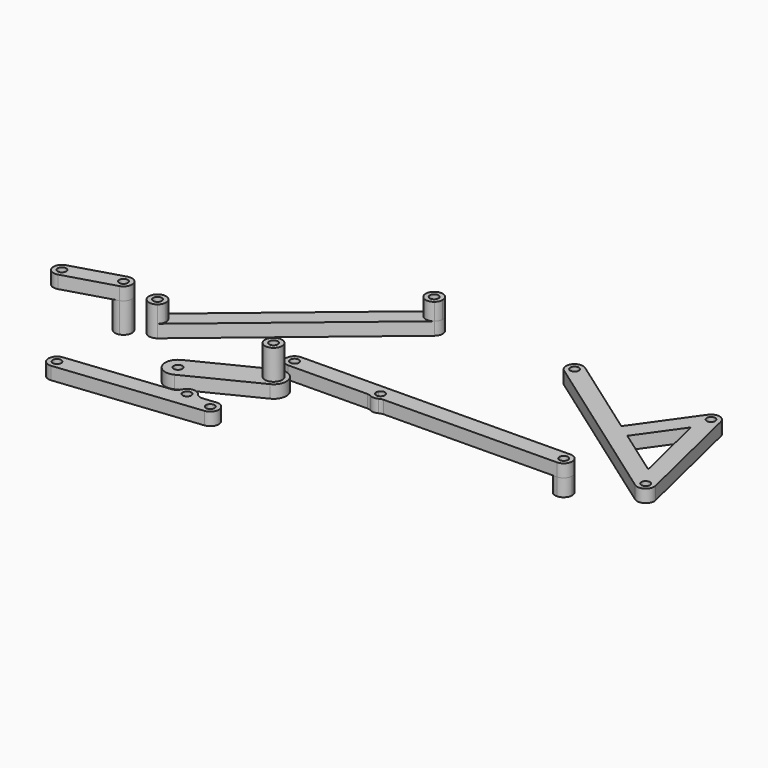
from build123d import *
from build123d import SkipClean  # not in build123d's __all__

# Parameters (mm, degrees)
F1_DEPTH  = 7.5
F2_R      = 5
F4_DEPTH  = 7.5
F5_R      = 5
F7_DEPTH  = 7.5
F8_R      = 2.5
F9_DEPTH  = 7.5
F11_DEPTH = 7.5
F12_R     = 2.5
F13_DEPTH = 10
F14_R     = 2.5
F15_DEPTH = 10
F16_R     = 2.5
F17_DEPTH = 17.5
F18_R     = 2.5
F19_DEPTH = 10
F20_R     = 5
F20_R_2   = 2.5
F21_DEPTH = 17.5


with BuildPart() as f1:
    # F0 (on Top) → F1 (new body)
    with BuildSketch(Plane.XY):
        with BuildLine():
            ThreePointArc((-1.6252031285, -41.1984268842), (-3.9906722267, -43.6948045472), (-6.6107242777, -41.4670988347))
            Line((-6.6107242777, -41.4670988347), (-14.4692804683, -42.316568018))
            ThreePointArc((-14.4692804683, -42.316568018), (-15.5453055293, -45.9890101187), (-18.9029788583, -47.8249542167))
            Line((-18.9029788583, -47.8249542167), (-3.5878592274, -46.1694691825))
            ThreePointArc((-3.5878592274, -46.1694691825), (0.8458391698, -40.661082983), (-4.6625470297, -36.2273845858))
            Line((-4.6625470297, -36.2273845858), (-15.3535819474, -37.3830300351))
            Line((-15.3535819474, -37.3830300351), (-15.0474170603, -39.0658729224))
            Line((-15.0474170603, -39.0658729224), (-6.5788708842, -40.7193501214))
            ThreePointArc((-6.5788708842, -40.7193501214), (-3.8845471388, -38.7100369038), (-1.6252031285, -41.1984268842))
        make_face()
        with BuildLine():
            ThreePointArc((-18.9029788583, -47.8249542167), (-15.5453055293, -45.9890101187), (-14.4692804683, -42.316568018))
            Line((-14.4692804683, -42.316568018), (-19.4403227667, -42.8539119191))
            Line((-19.4403227667, -42.8539119191), (-24.4243816475, -43.3926628454))
            Line((-24.4243816475, -43.3926628454), (-24.3595727591, -43.7488865063))
            ThreePointArc((-24.3595727591, -43.7488865063), (-22.432622422, -46.8596756132), (-18.9029788583, -47.8249542167))
        make_face()
        with BuildLine():
            Line((-17.8630008002, -38.516132339), (-15.0474170603, -39.0658729224))
            Line((-15.0474170603, -39.0658729224), (-15.3535819474, -37.3830300351))
            Line((-15.3535819474, -37.3830300351), (-15.3974185634, -37.1420809891))
            ThreePointArc((-15.3974185634, -37.1420809891), (-20.9754157833, -33.0806403303), (-25.2989118261, -38.4580686356))
            Line((-25.2989118261, -38.4580686356), (-87.3721108551, -45.1678596456))
            ThreePointArc((-87.3721108551, -45.1678596456), (-91.8058092522, -50.6762458451), (-86.2974230527, -55.1099442423))
            Line((-86.2974230527, -55.1099442423), (-18.9029788583, -47.8249542167))
            ThreePointArc((-18.9029788583, -47.8249542167), (-22.432622422, -46.8596756132), (-24.3595727591, -43.7488865063))
            Line((-24.3595727591, -43.7488865063), (-24.4243816475, -43.3926628454))
            Line((-24.4243816475, -43.3926628454), (-84.3492458047, -49.8702299933))
            ThreePointArc((-84.3492458047, -49.8702299933), (-84.3383892909, -50.0043710421), (-84.3347669539, -50.1389019439))
            ThreePointArc((-84.3347669539, -50.1389019439), (-89.3246527435, -50.3635544639), (-84.3751419577, -49.6914146503))
            Line((-84.3751419577, -49.6914146503), (-25.2359185483, -38.9320301634))
            Line((-25.2359185483, -38.9320301634), (-22.7762935521, -38.4845428698))
            ThreePointArc((-22.7762935521, -38.4845428698), (-22.7985582034, -38.337428307), (-22.8120316405, -38.1892497802))
            ThreePointArc((-22.8120316405, -38.1892497802), (-20.5853405064, -35.5515344271), (-17.8464232598, -37.6524932574))
            ThreePointArc((-17.8464232598, -37.6524932574), (-17.8241183317, -37.8441997236), (-17.8166685559, -38.0370555762))
            ThreePointArc((-17.8166685559, -38.0370555762), (-17.8282785754, -38.2777115659), (-17.8630008002, -38.516132339))
        make_face()
        with BuildLine():
            Line((-84.3492458047, -49.8702299933), (-24.4243816475, -43.3926628454))
            Line((-24.4243816475, -43.3926628454), (-25.2359185483, -38.9320301634))
            Line((-25.2359185483, -38.9320301634), (-84.3751419577, -49.6914146503))
            ThreePointArc((-84.3751419577, -49.6914146503), (-84.3605779289, -49.7805882986), (-84.3492458047, -49.8702299933))
        make_face()
        with BuildLine():
            Line((-24.4243816475, -43.3926628454), (-19.4403227667, -42.8539119191))
            Line((-19.4403227667, -42.8539119191), (-19.8691812623, -40.4966805725))
            ThreePointArc((-19.8691812623, -40.4966805725), (-21.7394647701, -40.09269439), (-22.7762935521, -38.4845428698))
            Line((-22.7762935521, -38.4845428698), (-25.2359185483, -38.9320301634))
            Line((-25.2359185483, -38.9320301634), (-24.4243816475, -43.3926628454))
        make_face()
        with BuildLine():
            Line((-19.4403227667, -42.8539119191), (-14.4692804683, -42.316568018))
            ThreePointArc((-14.4692804683, -42.316568018), (-14.4919447166, -42.1372846285), (-14.5210727742, -41.958937332))
            Line((-14.5210727742, -41.958937332), (-15.0474170603, -39.0658729224))
            Line((-15.0474170603, -39.0658729224), (-17.8630008002, -38.516132339))
            ThreePointArc((-17.8630008002, -38.516132339), (-18.560303565, -39.8161514193), (-19.8691812623, -40.4966805725))
            Line((-19.8691812623, -40.4966805725), (-19.4403227667, -42.8539119191))
        make_face()
        with BuildLine():
            Line((-14.4692804683, -42.316568018), (-6.6107242777, -41.4670988347))
            ThreePointArc((-6.6107242777, -41.4670988347), (-6.6229378611, -41.0920257285), (-6.5788708842, -40.7193501214))
            Line((-6.5788708842, -40.7193501214), (-15.0474170603, -39.0658729224))
            Line((-15.0474170603, -39.0658729224), (-14.5210727742, -41.958937332))
            ThreePointArc((-14.5210727742, -41.958937332), (-14.4919447166, -42.1372846285), (-14.4692804683, -42.316568018))
        make_face()
    extrude(amount=F1_DEPTH)

    # F2
    f2_edges = [f1.edges().sort_by_distance(p)[0] for p in [
        (-15.353582, -37.38303, 3.75),
        (-25.298912, -38.458069, 3.75),
    ]]
    fillet(f2_edges, radius=F2_R)


with BuildPart() as f4:
    # F3 (on Top) → F4 (new body)
    with BuildSketch(Plane.XY):
        with BuildLine():
            ThreePointArc((0.3729692735, 18.0101927138), (-4.6268408802, 18.0424809595), (0.3730047678, 18.0687030944))
            Line((0.3730047678, 18.0687030944), (43.7480600824, 18.5500000326))
            ThreePointArc((43.7480600824, 18.5500000326), (45.173207574, 22.1015652772), (48.6922749028, 23.6051696781))
            Line((48.6922749028, 23.6051696781), (-2.1823187693, 23.0406565959))
            ThreePointArc((-2.1823187693, 23.0406565959), (-7.1265335562, 17.9854869508), (-2.0713639111, 13.0412721639))
            Line((-2.0713639111, 13.0412721639), (45.5774592227, 13.5699915515))
            ThreePointArc((45.5774592227, 13.5699915515), (44.2716236478, 15.240737181), (43.7756797378, 17.3024445185))
            Line((43.7756797378, 17.3024445185), (43.7717936651, 17.4759705915))
            Line((43.7717936651, 17.4759705915), (0.3729692735, 18.0101927138))
        make_face()
        with BuildLine():
            ThreePointArc((48.6922749028, 23.6051696781), (45.173207574, 22.1015652772), (43.7480600824, 18.5500000326))
            Line((43.7480600824, 18.5500000326), (46.5634398285, 18.5812399617))
            ThreePointArc((46.5634398285, 18.5812399617), (48.7466876828, 19.9142362969), (50.9589766417, 18.6300135804))
            Line((50.9589766417, 18.6300135804), (53.7477634707, 18.66095843))
            Line((53.7477634707, 18.66095843), (53.746498958, 18.7174231321))
            ThreePointArc((53.746498958, 18.7174231321), (52.2235967035, 22.1997097401), (48.6922749028, 23.6051696781))
        make_face()
        with BuildLine():
            Line((46.2746157836, 17.445161855), (43.7717936651, 17.4759705915))
            Line((43.7717936651, 17.4759705915), (43.7756797378, 17.3024445185))
            ThreePointArc((43.7756797378, 17.3024445185), (44.2716236478, 15.240737181), (45.5774592227, 13.5699915515))
            Line((45.5774592227, 13.5699915515), (52.0559121057, 13.6418775586))
            ThreePointArc((52.0559121057, 13.6418775586), (53.3474796541, 15.3927117005), (53.773173057, 17.5263358594))
            Line((53.773173057, 17.5263358594), (51.2737997272, 17.4703630242))
            ThreePointArc((51.2737997272, 17.4703630242), (51.2742697249, 17.4423783605), (51.2744263974, 17.4143901889))
            ThreePointArc((51.2744263974, 17.4143901889), (48.7590402729, 14.9144375359), (46.2746157836, 17.445161855))
        make_face()
        with BuildLine():
            Line((154.1643564376, 24.775505705), (48.6922749028, 23.6051696781))
            ThreePointArc((48.6922749028, 23.6051696781), (52.2235967035, 22.1997097401), (53.746498958, 18.7174231321))
            Line((53.746498958, 18.7174231321), (53.7477634707, 18.66095843))
            Line((53.7477634707, 18.66095843), (151.7199877587, 19.7480747745))
            ThreePointArc((151.7199877587, 19.7480747745), (154.205964296, 22.2757750157), (156.7198338667, 19.775813489))
            ThreePointArc((156.7198338667, 19.775813489), (154.2478220383, 17.2759701615), (151.7204605369, 19.7198406538))
            Line((151.7204605369, 19.7198406538), (53.773173057, 17.5263358594))
            ThreePointArc((53.773173057, 17.5263358594), (53.3474796541, 15.3927117005), (52.0559121057, 13.6418775586))
            Line((52.0559121057, 13.6418775586), (154.2753112958, 14.776121273))
            ThreePointArc((154.2753112958, 14.776121273), (159.2195260827, 19.8312909181), (154.1643564376, 24.775505705))
        make_face()
        with BuildLine():
            Line((52.0559121057, 13.6418775586), (45.5774592227, 13.5699915515))
            ThreePointArc((45.5774592227, 13.5699915515), (48.8299038265, 12.4146979729), (52.0559121057, 13.6418775586))
        make_face()
        with BuildLine():
            Line((151.7199877587, 19.7480747745), (53.7477634707, 18.66095843))
            Line((53.7477634707, 18.66095843), (53.773173057, 17.5263358594))
            Line((53.773173057, 17.5263358594), (151.7204605369, 19.7198406538))
            ThreePointArc((151.7204605369, 19.7198406538), (151.7201842836, 19.7339570466), (151.7199877587, 19.7480747745))
        make_face()
        with BuildLine():
            Line((46.5634398285, 18.5812399617), (43.7480600824, 18.5500000326))
            ThreePointArc((43.7480600824, 18.5500000326), (43.7484531322, 18.5217645769), (43.7490056388, 18.4935317913))
            Line((43.7490056388, 18.4935317913), (43.7717936651, 17.4759705915))
            Line((43.7717936651, 17.4759705915), (46.2746157836, 17.445161855))
            ThreePointArc((46.2746157836, 17.445161855), (46.3515002965, 18.0303683622), (46.5634398285, 18.5812399617))
        make_face()
        with BuildLine():
            Line((43.7480600824, 18.5500000326), (0.3730047678, 18.0687030944))
            ThreePointArc((0.3730047678, 18.0687030944), (0.3731201865, 18.0548339506), (0.3731586598, 18.0409643799))
            ThreePointArc((0.3731586598, 18.0409643799), (0.3731113128, 18.0255782555), (0.3729692735, 18.0101927138))
            Line((0.3729692735, 18.0101927138), (43.7717936651, 17.4759705915))
            Line((43.7717936651, 17.4759705915), (43.7490056388, 18.4935317913))
            ThreePointArc((43.7490056388, 18.4935317913), (43.7484531322, 18.5217645769), (43.7480600824, 18.5500000326))
        make_face()
        with BuildLine():
            Line((53.7477634707, 18.66095843), (50.9589766417, 18.6300135804))
            ThreePointArc((50.9589766417, 18.6300135804), (51.1870976069, 18.0693845666), (51.2737997272, 17.4703630242))
            Line((51.2737997272, 17.4703630242), (53.773173057, 17.5263358594))
            Line((53.773173057, 17.5263358594), (53.7477634707, 18.66095843))
        make_face()
    extrude(amount=F4_DEPTH)

    # F5
    f5_edges = [f4.edges().sort_by_distance(p)[0] for p in [
        (45.577459, 13.569992, 3.75),
        (52.055912, 13.641878, 3.75),
    ]]
    fillet(f5_edges, radius=F5_R)

    # F14 (on face) → F15 (join)
    with BuildSketch(Plane(origin=(0, 0, 0), x_dir=(1, 0, 0), z_dir=(0, 0, -1))):
        with BuildLine():
            ThreePointArc((154.2753112958, -14.776121273), (149.2201416507, -19.7203360599), (154.1643564376, -24.775505705))
            ThreePointArc((154.1643564376, -24.775505705), (157.7356988282, -23.3309075205), (159.2198338667, -19.775813489))
            ThreePointArc((159.2198338667, -19.775813489), (157.7749278982, -16.2599485275), (154.2753112958, -14.776121273))
        make_face()
        with Locations((154.2198338667, -19.775813489)):
            Circle(F14_R, mode=Mode.SUBTRACT)
    extrude(amount=F15_DEPTH)


with BuildPart() as f7:
    # F6 (on Top) → F7 (new body)
    with BuildSketch(Plane.XY):
        with BuildLine():
            ThreePointArc((23.0980938211, 88.9733356379), (23.7370777778, 96.0154730622), (16.6949403535, 96.6544570189))
            Line((16.6949403535, 96.6544570189), (-80.5939894362, 15.5522432611))
            ThreePointArc((-80.5939894362, 15.5522432611), (-81.2329733929, 8.5101058368), (-74.1908359686, 7.8711218801))
            Line((-74.1908359686, 7.8711218801), (23.0980938211, 88.9733356379))
        make_face()
        with BuildLine():
            ThreePointArc((-74.8924127024, 11.7116825706), (-79.743019099, 10.8604190577), (-75.4721323571, 13.3124709375))
            ThreePointArc((-75.4721323571, 13.3124709375), (-75.0418063058, 12.5629460835), (-74.8924127024, 11.7116825706))
        make_face(mode=Mode.SUBTRACT)
        with BuildLine():
            ThreePointArc((22.3965170873, 92.8138963284), (20.7477806002, 90.4632899318), (17.976236742, 91.2131079615))
            ThreePointArc((17.976236742, 91.2131079615), (19.0452535744, 95.164502725), (22.3965170873, 92.8138963284))
        make_face(mode=Mode.SUBTRACT)
    extrude(amount=F7_DEPTH)

    # F12 (on face) → F13 (join)
    with BuildSketch(Plane.XY.offset(7.5)):
        with BuildLine():
            ThreePointArc((24.8965170873, 92.8138963284), (22.016908128, 97.3420241794), (16.6949403535, 96.6544570189))
            ThreePointArc((16.6949403535, 96.6544570189), (16.0559563968, 89.6123195946), (23.0980938211, 88.9733356379))
            ThreePointArc((23.0980938211, 88.9733356379), (24.4246449382, 90.6935052877), (24.8965170873, 92.8138963284))
        make_face()
        with Locations((19.8965170873, 92.8138963284)):
            Circle(F12_R, mode=Mode.SUBTRACT)
    extrude(amount=F13_DEPTH)

    # F18 (on face) → F19 (join)
    with BuildSketch(Plane.XY.offset(7.5)):
        with BuildLine():
            ThreePointArc((-80.5939894362, 15.5522432611), (-81.2329733929, 8.5101058368), (-74.1908359686, 7.8711218801))
            ThreePointArc((-74.1908359686, 7.8711218801), (-72.8642848515, 9.5912915299), (-72.3924127024, 11.7116825706))
            ThreePointArc((-72.3924127024, 11.7116825706), (-75.2720216617, 16.2398104216), (-80.5939894362, 15.5522432611))
        make_face()
        with Locations((-77.3924127024, 11.7116825706)):
            Circle(F18_R, mode=Mode.SUBTRACT)
    extrude(amount=F19_DEPTH)


with BuildPart() as f7b:
    # F6 (on Top) → F7, piece 2 (new body)
    with BuildSketch(Plane.XY):
        with BuildLine():
            ThreePointArc((-143.2768418385, 27.0090536761), (-146.6393941629, 20.7886644707), (-140.4190049575, 17.4261121464))
            Line((-140.4190049575, 17.4261121464), (-111.2633845005, 26.1209379651))
            ThreePointArc((-111.2633845005, 26.1209379651), (-107.9008321762, 32.3413271705), (-114.1212213815, 35.7038794948))
            Line((-114.1212213815, 35.7038794948), (-143.2768418385, 27.0090536761))
        make_face()
        with BuildLine():
            ThreePointArc((-139.347923398, 22.2175829113), (-144.3217199192, 21.8565693769), (-139.4521880156, 22.9320421315))
            ThreePointArc((-139.4521880156, 22.9320421315), (-139.3741268769, 22.5785964456), (-139.347923398, 22.2175829113))
        make_face(mode=Mode.SUBTRACT)
        with BuildLine():
            ThreePointArc((-110.192302941, 30.9124087299), (-112.3312894067, 28.4386122088), (-115.0880383234, 30.1979495097))
            ThreePointArc((-115.0880383234, 30.1979495097), (-113.0533164754, 33.3862052511), (-110.192302941, 30.9124087299))
        make_face(mode=Mode.SUBTRACT)
    extrude(amount=F7_DEPTH)

    # F16 (on face) → F17 (join)
    with BuildSketch(Plane(origin=(0, 0, 0), x_dir=(1, 0, 0), z_dir=(0, 0, -1))):
        with BuildLine():
            ThreePointArc((-111.2633845005, -26.1209379651), (-117.4837737059, -29.4834902894), (-114.1212213815, -35.7038794948))
            ThreePointArc((-114.1212213815, -35.7038794948), (-109.7043765867, -34.9214355571), (-107.692302941, -30.9124087299))
            ThreePointArc((-107.692302941, -30.9124087299), (-108.6832761138, -27.9244823756), (-111.2633845005, -26.1209379651))
        make_face()
        with Locations((-112.692302941, -30.9124087299)):
            Circle(F16_R, mode=Mode.SUBTRACT)
    with SkipClean():  # cleaning this boolean's faces spoils the solid; the shape is the same uncleaned
        extrude(amount=F17_DEPTH)


with BuildPart() as f9:
    # F8 (on Top) → F9 (new body)
    with BuildSketch(Plane.XY):
        with BuildLine():
            ThreePointArc((102.7963197006, 96.9999852765), (98.0322393826, 93.5173869112), (99.9046646538, 87.9210509443))
            Line((99.9046646538, 87.9210509443), (196.2528462269, 19.6149425153))
            ThreePointArc((196.2528462269, 19.6149425153), (195.002467233, 20.8934023144), (194.2819356808, 22.5300884078))
            Line((194.2819356808, 22.5300884078), (191.1861989539, 35.4650492124))
            Line((191.1861989539, 35.4650492124), (162.9887393202, 55.4556572728))
            Line((162.9887393202, 55.4556572728), (154.8587189983, 61.2194406735))
            Line((154.8587189983, 61.2194406735), (105.6881911573, 96.078919611))
            ThreePointArc((105.6881911573, 96.078919611), (104.3138295391, 96.7641738006), (102.7963197006, 96.9999852765))
        make_face()
        with Locations((102.7964279056, 91.9999852777)):
            Circle(F8_R, mode=Mode.SUBTRACT)
        with BuildLine():
            ThreePointArc((194.2819356808, 22.5300884078), (195.002467233, 20.8934023144), (196.2528462269, 19.6149425153))
            ThreePointArc((196.2528462269, 19.6149425153), (201.9450840129, 19.551734603), (204.0072832766, 24.8576652895))
            ThreePointArc((204.0072832766, 24.8576652895), (203.2867517243, 26.4943513829), (202.0363727305, 27.772811182))
            Line((202.0363727305, 27.772811182), (191.1861989539, 35.4650492124))
            Line((191.1861989539, 35.4650492124), (194.2819356808, 22.5300884078))
        make_face()
        with Locations((199.1446094787, 23.6938768487)):
            Circle(F8_R, mode=Mode.SUBTRACT)
        with BuildLine():
            ThreePointArc((202.0363727305, 27.772811182), (203.2867517243, 26.4943513829), (204.0072832766, 24.8576652895))
            Line((204.0072832766, 24.8576652895), (187.6591016847, 93.165504998))
            ThreePointArc((187.6591016847, 93.165504998), (187.6552696367, 90.8220314934), (186.5840700208, 88.737705671))
            Line((186.5840700208, 88.737705671), (180.4927420797, 80.1456721912))
            Line((180.4927420797, 80.1456721912), (191.1861989539, 35.4650492124))
            Line((191.1861989539, 35.4650492124), (202.0363727305, 27.772811182))
        make_face()
        with BuildLine():
            Line((178.5286055467, 94.6066527316), (154.8587189983, 61.2194406735))
            Line((154.8587189983, 61.2194406735), (162.9887393202, 55.4556572728))
            Line((162.9887393202, 55.4556572728), (180.4927420797, 80.1456721912))
            Line((180.4927420797, 80.1456721912), (177.9337540889, 90.8379281163))
            ThreePointArc((177.9337540889, 90.8379281163), (177.8575706062, 92.7812605018), (178.5286055467, 94.6066527316))
        make_face()
        with BuildLine():
            ThreePointArc((186.5840700208, 88.737705671), (187.6552696367, 90.8220314934), (187.6591016847, 93.165504998))
            ThreePointArc((187.6591016847, 93.165504998), (185.8932433182, 95.9272399852), (182.7963196819, 97.001716556))
            ThreePointArc((182.7963196819, 97.001716556), (180.6545031685, 96.5196982416), (178.9256257198, 95.1666637263))
            Line((178.9256257198, 95.1666637263), (178.5286055467, 94.6066527316))
            ThreePointArc((178.5286055467, 94.6066527316), (177.8575706062, 92.7812605018), (177.9337540889, 90.8379281163))
            Line((177.9337540889, 90.8379281163), (180.4927420797, 80.1456721912))
            Line((180.4927420797, 80.1456721912), (186.5840700208, 88.737705671))
        make_face()
        with Locations((182.7964278868, 92.0017165571)):
            Circle(F8_R, mode=Mode.SUBTRACT)
        with BuildLine():
            ThreePointArc((178.9256257198, 95.1666637263), (178.7174935535, 94.8934798089), (178.5286055467, 94.6066527316))
            Line((178.5286055467, 94.6066527316), (178.9256257198, 95.1666637263))
        make_face()
    extrude(amount=F9_DEPTH)


with BuildPart() as f11:
    # F10 (on Top) → F11 (new body)
    with BuildSketch(Plane.XY):
        with BuildLine():
            ThreePointArc((3.3541019662, -6.7082039325), (6.7082039325, 3.3541019662), (-3.3541019662, 6.7082039325))
            Line((-3.3541019662, 6.7082039325), (-43.3541019662, -13.2917960675))
            ThreePointArc((-43.3541019662, -13.2917960675), (-46.7082039325, -23.3541019662), (-36.6458980338, -26.7082039325))
            Line((-36.6458980338, -26.7082039325), (3.3541019662, -6.7082039325))
        make_face()
        with BuildLine():
            ThreePointArc((-37.5, -20), (-42.4331224737, -20.5743823014), (-37.7639320225, -18.8819660113))
            ThreePointArc((-37.7639320225, -18.8819660113), (-37.5668775263, -19.4256176986), (-37.5, -20))
        make_face(mode=Mode.SUBTRACT)
        with BuildLine():
            ThreePointArc((2.5, 0), (0.5743823014, -2.4331224737), (-2.2360679775, -1.1180339887))
            ThreePointArc((-2.2360679775, -1.1180339887), (-0.5743823014, 2.4331224737), (2.5, 0))
        make_face(mode=Mode.SUBTRACT)
    extrude(amount=F11_DEPTH)

    # F20 (on face) → F21 (join)
    with BuildSketch(Plane.XY.offset(7.5)):
        Circle(F20_R)
        Circle(F20_R_2, mode=Mode.SUBTRACT)
    extrude(amount=F21_DEPTH)


solid = Compound([f1.part, f4.part, f7.part, f7b.part, f9.part, f11.part])
